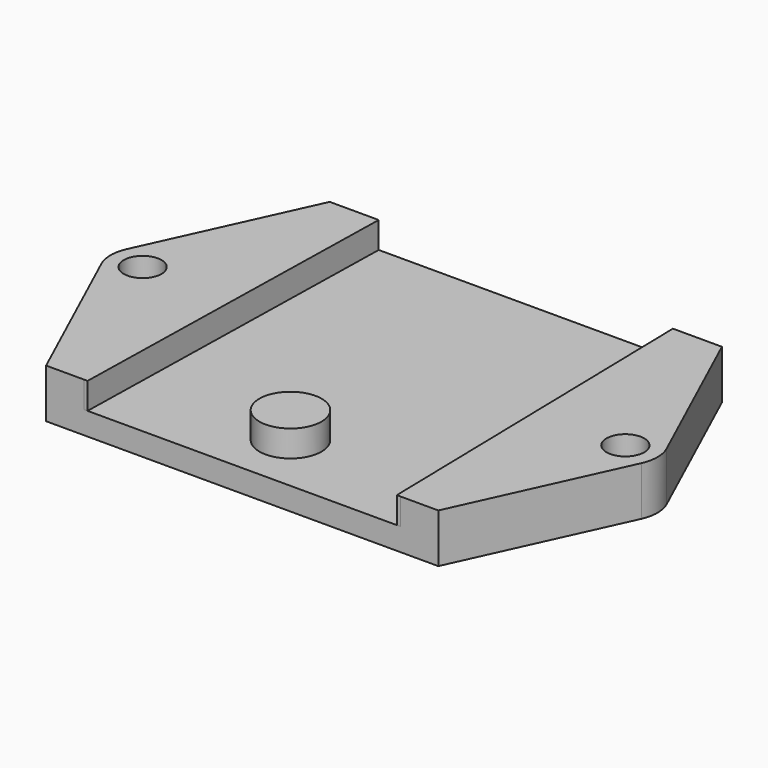
from build123d import *

# Parameters (mm, degrees)
F0_R     = 2.5
F0_R_2   = 4.125
F1_DEPTH = 6.5
F2_DEPTH = 3.5
F3_R     = 5
F4_DEPTH = 0.5
F5_DEPTH = 0.5


# Not quite as in the source:
# - a feature names something its author has since deleted; it is built from what else it names


with BuildPart() as f1:
    # F0 (on Top) → F1 (new body)
    with BuildSketch(Plane.XY):
        Polygon((-16.7020111382, 19.4748209119), (-22.7020111382, 19.4748209119), (-33.4520111382, -4.0251790881), (-22.7020111382, -27.5251790881), (-17.7020111382, -27.5251790881), align=None)
        with Locations((-28.7020111382, -4.0251790881)):
            Circle(F0_R, mode=Mode.SUBTRACT)
        Polygon((23.2979888618, 19.4748209119), (-16.7020111382, 19.4748209119), (-17.7020111382, -27.5251790881), (24.2979888618, -27.5251790881), align=None)
        with Locations((3.2979888618, -19.5251790881)):
            Circle(F0_R_2, mode=Mode.SUBTRACT)
        Polygon((29.2979888618, 19.4748209119), (23.2979888618, 19.4748209119), (24.2979888618, -27.5251790881), (29.2979888618, -27.5251790881), (40.0479888618, -4.0251790881), align=None)
        with Locations((35.2979888618, -4.0251790881)):
            Circle(F0_R, mode=Mode.SUBTRACT)
        with Locations((3.2979888618, -19.5251790881)):
            Circle(F0_R_2)
    extrude(amount=-F1_DEPTH)

    # F0 (on Top) → F2 (cut)
    with BuildSketch(Plane.XY):
        Polygon((23.2979888618, 19.4748209119), (-16.7020111382, 19.4748209119), (-17.7020111382, -27.5251790881), (24.2979888618, -27.5251790881), align=None)
        with Locations((3.2979888618, -19.5251790881)):
            Circle(F0_R_2, mode=Mode.SUBTRACT)
    extrude(amount=-F2_DEPTH, mode=Mode.SUBTRACT)

    # F3
    f3_edges = [f1.edges().sort_by_distance(p)[0] for p in [
        (-33.452011, -4.025179, -3.25),
        (40.047989, -4.025179, -3.25),
    ]]
    fillet(f3_edges, radius=F3_R)

    # F4 (add): a face of the model
    f4_faces = [f1.faces().sort_by_distance(p)[0] for p in [
        (-17.2020111382, -4.0251790881, -1.75),
    ]]
    extrude(f4_faces, amount=F4_DEPTH)

    # F5 (add): a face of the model
    f5_faces = [f1.faces().sort_by_distance(p)[0] for p in [
        (23.7979888618, -4.0251790881, -1.75),
    ]]
    extrude(f5_faces, amount=F5_DEPTH)


solid = f1.part
